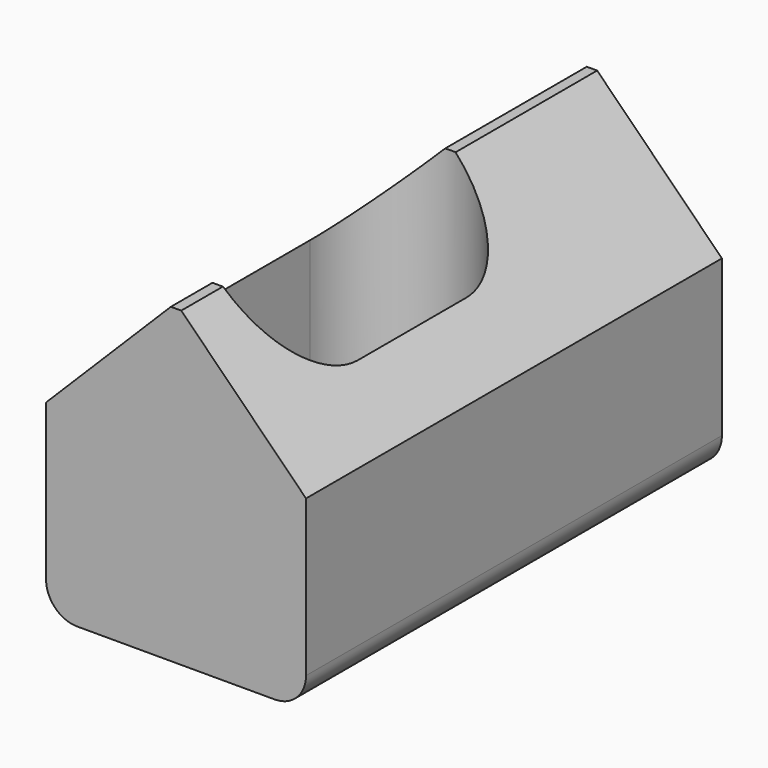
from build123d import *

# Parameters (mm, degrees)
F0_W        = 6.35
F0_H        = 12.7
F1_DEPTH    = 7.62
F3_DEPTH    = 6.35
F4_T1_DEPTH = 28.3769794946
F5_R        = 0.762


# Not quite as in the source:
# - a fillet or chamfer that OpenCascade refuses, or shapes differently, is made with other operations: its cross-section is extruded or revolved along the edge and cut away or added
# - a feature names something its author has since deleted; it is built from what else it names


with BuildPart() as f1:
    # F0 (on Top) → F1 (new body)
    with BuildSketch(Plane.XY):
        with Locations((-47.625, -6.35)):
            Rectangle(F0_W, F0_H)
    extrude(amount=F1_DEPTH)

    # F2 (on face) → F3 (cut)
    with BuildSketch(Plane.XY.offset(7.62)):
        with BuildLine():
            ThreePointArc((-45.72, -6.223), (-47.625, -4.318), (-49.53, -6.223))
            Line((-49.53, -6.223), (-49.53, -9.525))
            ThreePointArc((-49.53, -9.525), (-47.625, -11.43), (-45.72, -9.525))
            Line((-45.72, -9.525), (-45.72, -6.223))
        make_face()
    extrude(amount=-F3_DEPTH, mode=Mode.SUBTRACT)

    # F4: chamfer of 3.048 on 2 edges, made by hand

    # F4_s2 → F4_t1 (cut)
    with BuildSketch(Plane.XZ.offset(-7.8384897473)):
        Polygon((-50.8, 4.572), (-47.752, 7.62), (-50.8, 7.62), align=None)
        Polygon((-44.45, 4.572), (-47.498, 7.62), (-44.45, 7.62), align=None)
    extrude(amount=F4_T1_DEPTH, mode=Mode.SUBTRACT)

    # F5
    f5_edges = [f1.edges().sort_by_distance(p)[0] for p in [
        (-50.8, -6.35, 0),
        (-44.45, -6.35, 0),
    ]]
    fillet(f5_edges, radius=F5_R)


solid = f1.part
